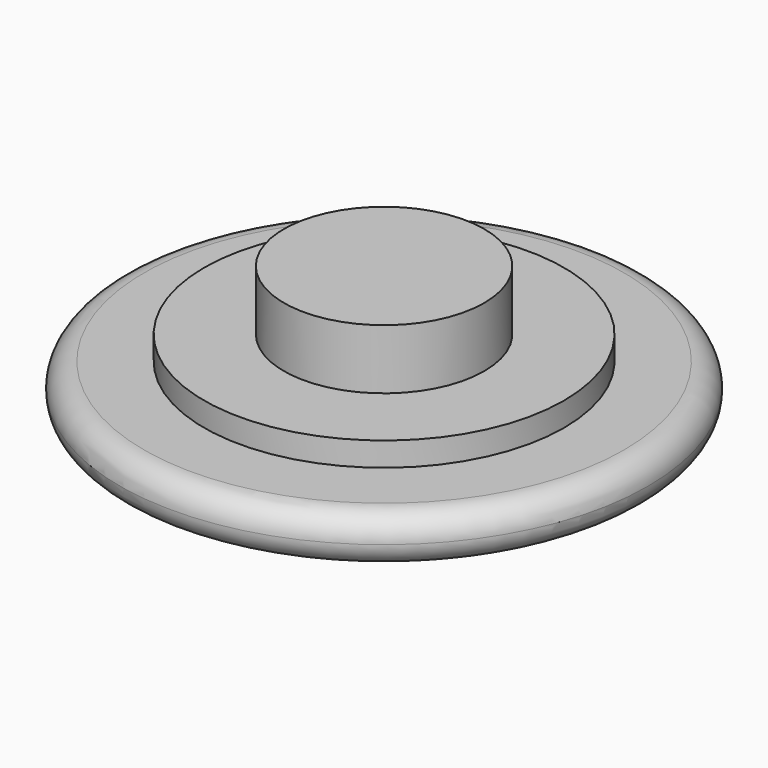
from build123d import *

# Parameters (mm, degrees)
F0_R         = 11
F0_R_2       = 7.5
F1_DEPTH     = 2
F0_R_3       = 4.175
F2_DEPTH     = 3
F3_DEPTH     = 5.5
F4_R         = 0.99999
F5_TEXT_SIZE = 6.4748338239
F6_DEPTH     = 1


# Not quite as in the source:
# - a fillet or chamfer is up to 0.001 mm smaller than in the source, because OpenCascade refuses the exact size
# - Text() gives the source's letters only with a copy of the font that has no kerning and outlines rounded to 1/6400 em; it was checked with that copy


with BuildPart() as f1:
    # F0 (on Top) → F1 (new body)
    with BuildSketch(Plane.XY):
        Circle(F0_R)
        Circle(F0_R_2, mode=Mode.SUBTRACT)
    extrude(amount=F1_DEPTH)

    # F0 (on Top) → F2 (join)
    with BuildSketch(Plane.XY):
        Circle(F0_R_2)
        Circle(F0_R_3, mode=Mode.SUBTRACT)
    extrude(amount=F2_DEPTH)

    # F0 (on Top) → F3 (join)
    with BuildSketch(Plane.XY):
        Circle(F0_R_3)
    extrude(amount=F3_DEPTH)

    # F4 (radius 1 in the source; OpenCascade refuses exactly that, so slightly less here)
    f4_edges = [f1.edges().sort_by_distance(p)[0] for p in [
        (-11, 0, 2),
        (-11, 0, 0),
    ]]
    fillet(f4_edges, radius=F4_R)

    # F5 (on face) → F6 (cut)
    with BuildSketch(Plane(origin=(0, 0, 0), x_dir=(1, 0, 0), z_dir=(0, 0, -1))):
        with Locations((-9.8412733985, -1.7746373983)):
            Text('Noelle', F5_TEXT_SIZE, font='Open Sans', text_align=(TextAlign.LEFT, TextAlign.BOTTOM))
    extrude(amount=-F6_DEPTH, mode=Mode.SUBTRACT)


solid = f1.part
